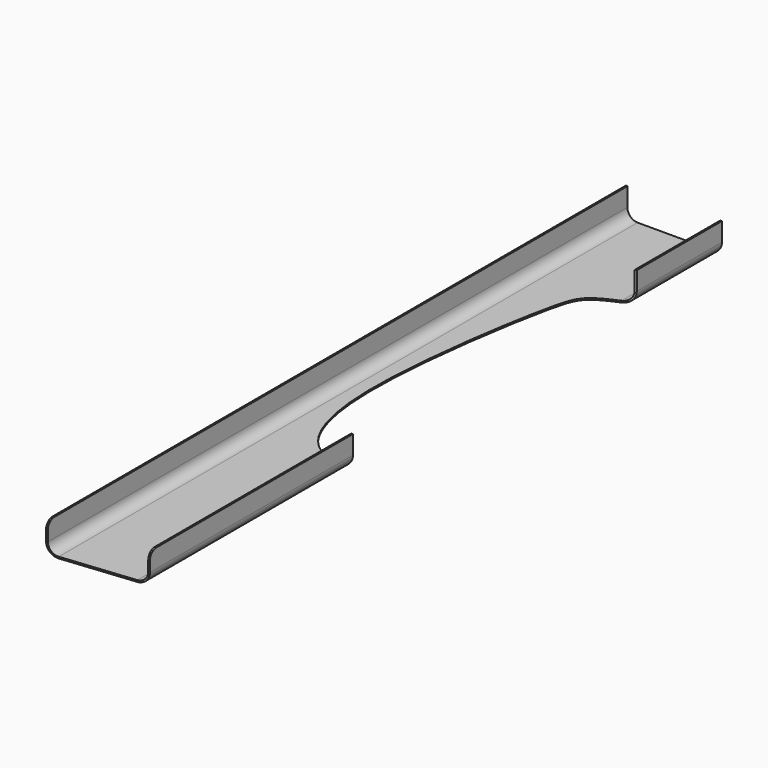
from build123d import *

# Parameters (mm, degrees)
F1_DEPTH      = 454.025
F3_DEPTH      = 19.051
F3_DEPTH_BACK = 686
F5_DEPTH      = 687
F5_DEPTH_BACK = 19.051
F6_R          = 5.08


# Not quite as in the source:
# - an extrude ends at something that could not be found from the text; its depth is read off the source's solid


with BuildPart() as f1:
    # F0 (on Front) → F1 (new body)
    with BuildSketch(Plane.XZ):
        with BuildLine():
            Line((29.083, 19.05), (29.083, 7.366))
            ThreePointArc((29.083, 7.366), (27.2231280605, 2.8758719395), (22.733, 1.016))
            Line((22.733, 1.016), (0, 1.016))
            Line((0, 1.016), (-22.733, 1.016))
            ThreePointArc((-22.733, 1.016), (-27.2231280605, 2.8758719395), (-29.083, 7.366))
            Line((-29.083, 7.366), (-29.083, 19.05))
            Line((-29.083, 19.05), (-30.099, 19.05))
            Line((-30.099, 19.05), (-30.099, 7.366))
            ThreePointArc((-30.099, 7.366), (-27.9415485502, 2.1574514498), (-22.733, 0))
            Line((-22.733, 0), (0, 0))
            Line((0, 0), (22.733, 0))
            ThreePointArc((22.733, 0), (27.9415485502, 2.1574514498), (30.099, 7.366))
            Line((30.099, 7.366), (30.099, 19.05))
            Line((30.099, 19.05), (29.083, 19.05))
        make_face()
    extrude(amount=-F1_DEPTH)

    # F2 (on face) → F3 (cut, two sides)
    with BuildSketch(Plane(origin=(0, 0, 0), x_dir=(1, 0, 0), z_dir=(0, 0, -1))) as f3_sk:
        Polygon((30.6164417416, -6.2488044892), (30.6164417416, 0), (-30.9091024101, 0), align=None)
    extrude(amount=-F3_DEPTH, mode=Mode.SUBTRACT)
    extrude(f3_sk.sketch, amount=F3_DEPTH_BACK, mode=Mode.SUBTRACT)

    # F4 (on Top) → F5 (cut, two sides)
    with BuildSketch(Plane.XY) as f5_sk:
        with BuildLine():
            Line((62.3281411827, 387.35), (30.0085749477, 387.35))
            add(Edge.make_bspline(
                [(30.0085749477, 165.1), (25.391612917, 164.5890872008), (15.3825161545, 163.4814810281), (-5.0321407016, 175.2210203018), (-21.9793035432, 229.6347611818), (-1.9935882921, 356.8923129343), (5.9717389451, 377.9788071194), (21.8185822716, 384.1569840369), (30.0085749477, 387.35)],
                knots=[0, 0, 0, 0, 0.1027234154, 0.2226937536, 0.4288641549, 0.7409489277, 0.8661167817, 1, 1, 1, 1], degree=3))
            Line((30.0085749477, 165.1), (62.3281411827, 165.9812778234))
            Line((62.3281411827, 165.9812778234), (62.3281411827, 387.35))
        make_face()
    extrude(amount=-F5_DEPTH, mode=Mode.SUBTRACT)
    extrude(f5_sk.sketch, amount=F5_DEPTH_BACK, mode=Mode.SUBTRACT)

    # F6
    f6_edges = [f1.edges().sort_by_distance(p)[0] for p in [
        (-29.591, 0.133872, 19.05),
        (29.591, 6.144656, 19.05),
    ]]
    fillet(f6_edges, radius=F6_R)


solid = f1.part
